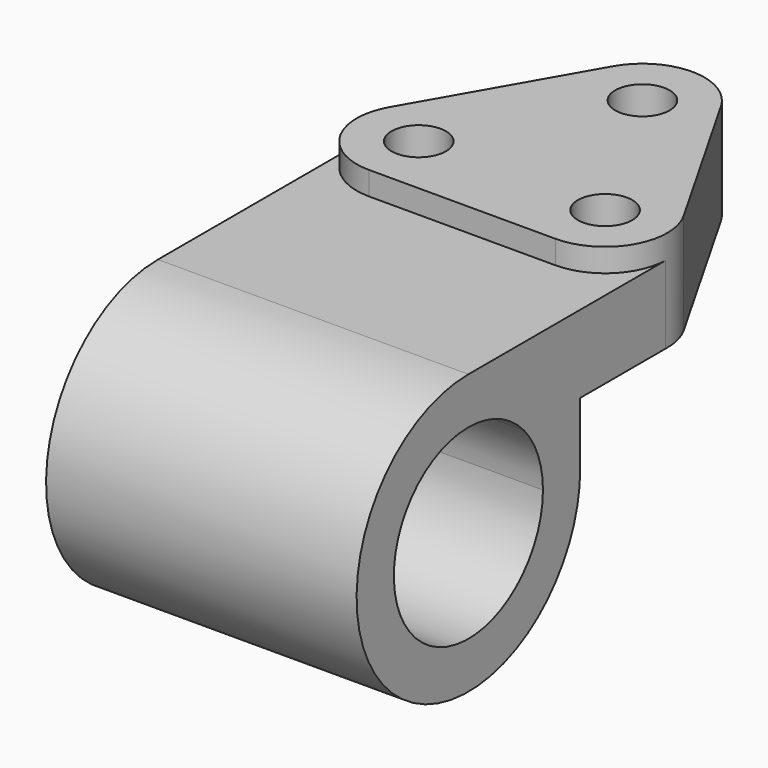
from build123d import *

# Parameters (mm, degrees)
F0_R          = 5.5626
F1_DEPTH      = 20.6502
F2_W          = 63.493296
F2_H          = 50.8
F3_DEPTH      = 15.875
F4_DEPTH      = 20.6512
F6_DEPTH      = 50.793296
F6_DEPTH_BACK = 12.7
F7_DEPTH      = 12.701
F7_DEPTH_BACK = 50.801
F8_DEPTH      = 23.8125
F9_DEPTH      = 14.2875


with BuildPart() as f1:
    # F0 (on Top) → F1 (new body)
    with BuildSketch(Plane.XY):
        with BuildLine():
            Line((8.022279, 52.349355), (-11.027721, 18.999155))
            ThreePointArc((-11.027721, 18.999155), (-10.983835, 6.324628), (0, 0))
            Line((0, 0), (38.1, 0))
            ThreePointArc((38.1, 0), (49.083835, 6.324628), (49.127721, 18.999155))
            Line((49.127721, 18.999155), (30.077721, 52.349355))
            ThreePointArc((30.077721, 52.349355), (19.05, 58.7502), (8.022279, 52.349355))
        make_face()
        with Locations((0, 12.7)):
            Circle(F0_R, mode=Mode.SUBTRACT)
        with Locations((38.1, 12.7)):
            Circle(F0_R, mode=Mode.SUBTRACT)
        with Locations((19.05, 46.0502)):
            Circle(F0_R, mode=Mode.SUBTRACT)
    extrude(amount=F1_DEPTH)

    # F2 (on Top) → F3 (join)
    with BuildSketch(Plane.XY):
        with Locations((19.046648, -12.7)):
            Rectangle(F2_W, F2_H)
    extrude(amount=F3_DEPTH)

    # F0 (on Top) → F4 (cut, through all)
    with BuildSketch(Plane.XY):
        with Locations((0, 12.7)):
            Circle(F0_R)
        with Locations((38.1, 12.7)):
            Circle(F0_R)
    extrude(amount=F4_DEPTH, mode=Mode.SUBTRACT)

    # F5 (on Right) → F6 (join, two sides)
    with BuildSketch(Plane.YZ) as f6_sk:
        with BuildLine():
            Line((-38.1, 6.35), (-38.1, 15.875))
            ThreePointArc((-38.1, 15.875), (-65.572384, -20.561217), (-22.984243, -36.949629))
            ThreePointArc((-22.984243, -36.949629), (-13.115371, -26.567189), (-9.525, -12.7))
            Line((-9.525, -12.7), (-9.525, 0))
            Line((-9.525, 0), (-23.900968, 0))
            ThreePointArc((-23.900968, 0), (-20.304017, -5.902539), (-19.05, -12.7))
            ThreePointArc((-19.05, -12.7), (-51.570384, -26.170384), (-38.1, 6.35))
        make_face()
    extrude(amount=F6_DEPTH)
    extrude(f6_sk.sketch, amount=-F6_DEPTH_BACK)

    # F5 (on Right) → F7 (cut, two sides)
    with BuildSketch(Plane.YZ) as f7_sk:
        with BuildLine():
            ThreePointArc((-23.900968, 0), (-30.32287, 4.690191), (-38.1, 6.35))
            ThreePointArc((-38.1, 6.35), (-51.570384, -26.170384), (-19.05, -12.7))
            ThreePointArc((-19.05, -12.7), (-20.304017, -5.902539), (-23.900968, 0))
        make_face()
    extrude(amount=-F7_DEPTH, mode=Mode.SUBTRACT)
    extrude(f7_sk.sketch, amount=F7_DEPTH_BACK, mode=Mode.SUBTRACT)

    # F5 (on Right) → F8 (join)
    with BuildSketch(Plane.YZ):
        with BuildLine():
            ThreePointArc((-9.525, -12.7), (-13.115371, -26.567189), (-22.984243, -36.949629))
            Line((-22.984243, -36.949629), (36.292628, 0))
            Line((36.292628, 0), (12.28739, 0))
            Line((12.28739, 0), (-9.525, 0))
            Line((-9.525, 0), (-9.525, -12.7))
        make_face()
    extrude(amount=F8_DEPTH)

    # F5 (on Right) → F9 (cut)
    with BuildSketch(Plane.YZ):
        with BuildLine():
            ThreePointArc((-9.525, -12.7), (-13.115371, -26.567189), (-22.984243, -36.949629))
            Line((-22.984243, -36.949629), (36.292628, 0))
            Line((36.292628, 0), (12.28739, 0))
            Line((12.28739, 0), (-9.525, 0))
            Line((-9.525, 0), (-9.525, -12.7))
        make_face()
    extrude(amount=F9_DEPTH, mode=Mode.SUBTRACT)


solid = f1.part
